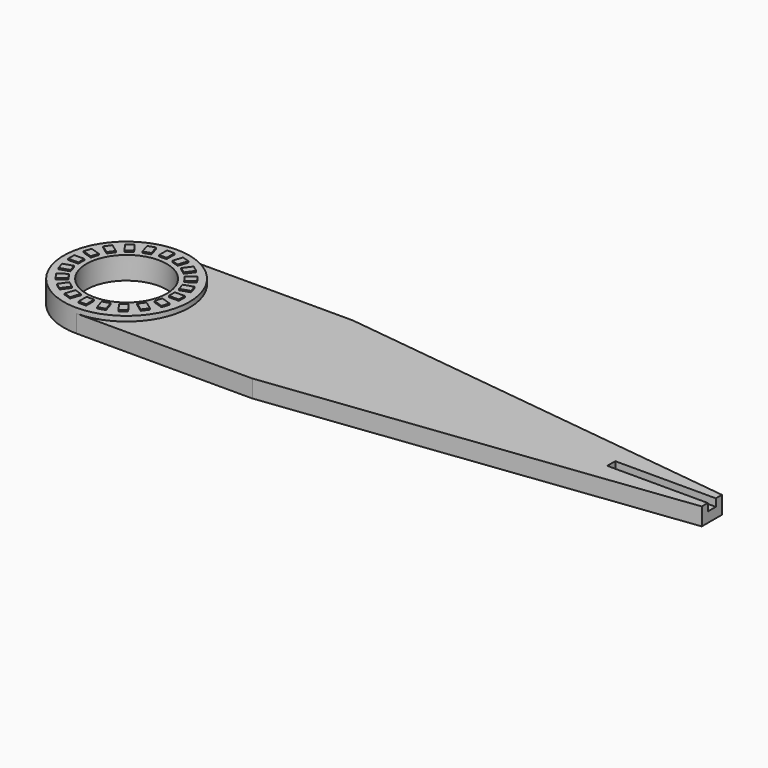
from build123d import *

# Parameters (mm, degrees)
F0_R         = 8
F1_DEPTH     = 3.5
F2_R         = 12.5
F2_R_2       = 8
F3_DEPTH     = 1
F4_W         = 1.5
F4_H         = 2
F4_W_2       = 2
F4_H_2       = 1.5
F5_DEPTH     = 0.25
F6_W         = 20
F6_H         = 2
F7_DEPTH     = 1.5
F8_TEXT_SIZE = 12.8578142418
F9_DEPTH     = 1


# Not quite as in the source:
# - Text() gives the source's letters only with a copy of the font that has no kerning and outlines rounded to 1/6400 em; it was checked with that copy


with BuildPart() as f1:
    # F0 (on Top) → F1 (new body)
    with BuildSketch(Plane.XY):
        with BuildLine():
            ThreePointArc((0, -12.5), (8.8388347648, -8.8388347648), (12.5, 0))
            ThreePointArc((12.5, 0), (8.8388347648, 8.8388347648), (0, 12.5))
            ThreePointArc((0, 12.5), (-12.5, 0), (0, -12.5))
        make_face()
        Circle(F0_R, mode=Mode.SUBTRACT)
        with BuildLine():
            ThreePointArc((0, 12.5), (8.8388347648, 8.8388347648), (12.5, 0))
            ThreePointArc((12.5, 0), (8.8388347648, -8.8388347648), (0, -12.5))
            Line((0, -12.5), (35, -12.5))
            Line((35, -12.5), (116.3887844346, -2.5067138408))
            Line((116.3887844346, -2.5067138408), (116.3887844346, 2.5067138408))
            Line((116.3887844346, 2.5067138408), (35, 12.5))
            Line((35, 12.5), (0, 12.5))
        make_face()
    extrude(amount=F1_DEPTH)

    # F2 (on face) → F3 (join)
    with BuildSketch(Plane.XY.offset(3.5)):
        Circle(F2_R)
        Circle(F2_R_2, mode=Mode.SUBTRACT)
    extrude(amount=F3_DEPTH)

    # F4 (on face) → F5 (join)
    with BuildSketch(Plane.XY.offset(4.5)):
        with Locations((0, 10)):
            Rectangle(F4_W, F4_H)
        Polygon((-2.0678605622, 8.7912713924), (-2.6858945509, 10.693384425), (-4.1124793253, 10.2298589335), (-3.4944453366, 8.3277459009), align=None)
        Polygon((-4.6833045249, 7.7219918886), (-5.8588750294, 9.3400258773), (-7.072400521, 8.4583479989), (-5.8968300164, 6.8403140102), align=None)
        Polygon((-6.8403140102, 5.8968300164), (-8.4583479989, 7.072400521), (-9.3400258773, 5.8588750294), (-7.7219918886, 4.6833045249), align=None)
        Polygon((-8.3277459009, 3.4944453366), (-10.2298589335, 4.1124793253), (-10.693384425, 2.6858945509), (-8.7912713924, 2.0678605622), align=None)
        with Locations((-10, 0)):
            Rectangle(F4_W_2, F4_H_2)
        Polygon((-8.7912713924, -2.0678605622), (-10.693384425, -2.6858945509), (-10.2298589335, -4.1124793253), (-8.3277459009, -3.4944453366), align=None)
        Polygon((-7.7219918886, -4.6833045249), (-9.3400258773, -5.8588750294), (-8.4583479989, -7.072400521), (-6.8403140102, -5.8968300164), align=None)
        Polygon((-5.8968300164, -6.8403140102), (-7.072400521, -8.4583479989), (-5.8588750294, -9.3400258773), (-4.6833045249, -7.7219918886), align=None)
        Polygon((-3.4944453366, -8.3277459009), (-4.1124793253, -10.2298589335), (-2.6858945509, -10.693384425), (-2.0678605622, -8.7912713924), align=None)
        with Locations((0, -10)):
            Rectangle(F4_W, F4_H)
        Polygon((2.0678605622, -8.7912713924), (2.6858945509, -10.693384425), (4.1124793253, -10.2298589335), (3.4944453366, -8.3277459009), align=None)
        Polygon((4.6833045249, -7.7219918886), (5.8588750294, -9.3400258773), (7.072400521, -8.4583479989), (5.8968300164, -6.8403140102), align=None)
        Polygon((6.8403140102, -5.8968300164), (8.4583479989, -7.072400521), (9.3400258773, -5.8588750294), (7.7219918886, -4.6833045249), align=None)
        Polygon((8.3277459009, -3.4944453366), (10.2298589335, -4.1124793253), (10.693384425, -2.6858945509), (8.7912713924, -2.0678605622), align=None)
        with Locations((10, 0)):
            Rectangle(F4_W_2, F4_H_2)
        Polygon((8.7912713924, 2.0678605622), (10.693384425, 2.6858945509), (10.2298589335, 4.1124793253), (8.3277459009, 3.4944453366), align=None)
        Polygon((7.7219918886, 4.6833045249), (9.3400258773, 5.8588750294), (8.4583479989, 7.072400521), (6.8403140102, 5.8968300164), align=None)
        Polygon((5.8968300164, 6.8403140102), (7.072400521, 8.4583479989), (5.8588750294, 9.3400258773), (4.6833045249, 7.7219918886), align=None)
        Polygon((3.4944453366, 8.3277459009), (4.1124793253, 10.2298589335), (2.6858945509, 10.693384425), (2.0678605622, 8.7912713924), align=None)
    extrude(amount=F5_DEPTH)

    # F6 (on face) → F7 (cut)
    with BuildSketch(Plane.XY.offset(3.5)):
        with Locations((106.3887844346, -0.0067138408)):
            Rectangle(F6_W, F6_H)
    extrude(amount=-F7_DEPTH, mode=Mode.SUBTRACT)


with BuildPart() as f9:
    # F8 (on face) → F9 (new body)
    with BuildSketch(Plane(origin=(0, 0, 0), x_dir=(1, 0, 0), z_dir=(0, 0, -1))):
        with Locations((13.6947203428, -3.9514261298)):
            Text('K.Hank', F8_TEXT_SIZE, font='Open Sans', font_style=FontStyle.ITALIC, text_align=(TextAlign.LEFT, TextAlign.BOTTOM))
    extrude(amount=F9_DEPTH)


solid = Compound([f1.part, f9.part])
